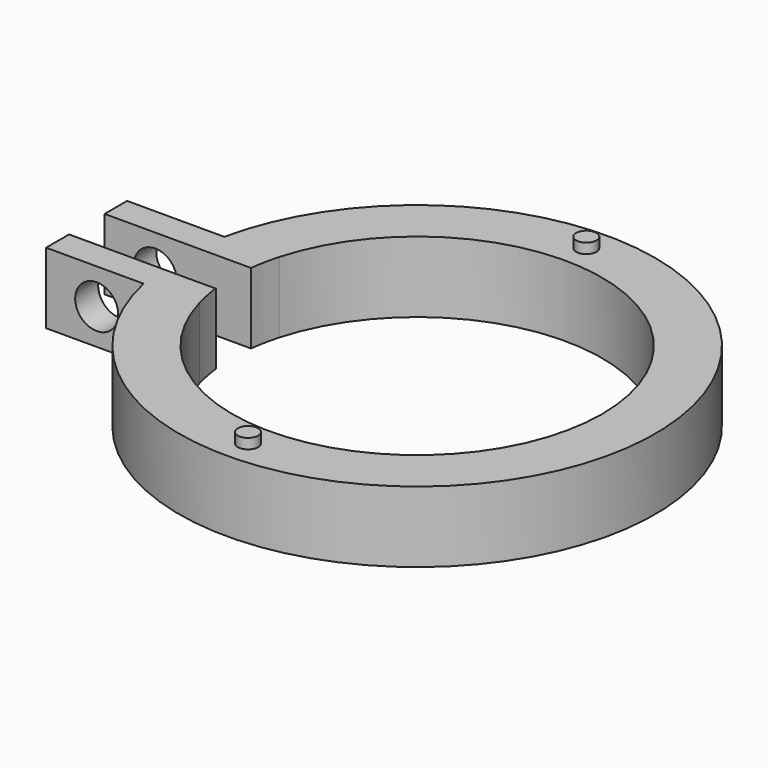
from build123d import *

# Parameters (mm, degrees)
F1_DEPTH = 7
F2_R     = 2.125
F3_DEPTH = 10
F4_R     = 1
F5_DEPTH = 1


# Not quite as in the source:
# - a feature names something its author has since deleted; it is built from what else it names


with BuildPart() as f1:
    # F0 (on Top) → F1 (new body)
    with BuildSketch(Plane.XY):
        with BuildLine():
            ThreePointArc((-23.401635828, 2.1478921234), (-23.2315061267, 3.5421918479), (-22.9783775489, 4.9238364331))
            Line((-22.9783775489, 4.9238364331), (-32.5732277849, 4.9238364331))
            Line((-32.5732277849, 4.9238364331), (-32.5732277849, 2.1478921234))
            Line((-32.5732277849, 2.1478921234), (-23.401635828, 2.1478921234))
        make_face()
        with BuildLine():
            Line((-32.5732277849, -5.0761635669), (-22.9452078535, -5.0761635669))
            ThreePointArc((-22.9452078535, -5.0761635669), (-23.2124017724, -3.6652972535), (-23.3929275249, -2.2407458164))
            Line((-23.3929275249, -2.2407458164), (-32.5732277849, -2.2407458164))
            Line((-32.5732277849, -2.2407458164), (-32.5732277849, -5.0761635669))
        make_face()
        with BuildLine():
            ThreePointArc((-22.9452078535, -5.0761635669), (2.55319559, -23.3608902287), (23.5, 0))
            ThreePointArc((23.5, 0), (2.4756946097, 23.3692305436), (-22.9783775489, 4.9238364331))
            Line((-22.9783775489, 4.9238364331), (-17.5732277849, 4.9238364331))
            ThreePointArc((-17.5732277849, 4.9238364331), (2.4850646798, 18.080015308), (18.25, 0))
            ThreePointArc((18.25, 0), (2.4850646798, -18.080015308), (-17.5732277849, -4.9238364331))
            Line((-17.5732277849, -4.9238364331), (-17.5732277849, -5.0761635669))
            Line((-17.5732277849, -5.0761635669), (-22.9452078535, -5.0761635669))
        make_face()
        with BuildLine():
            Line((-17.5732277849, 4.9238364331), (-22.9783775489, 4.9238364331))
            ThreePointArc((-22.9783775489, 4.9238364331), (-23.2315061267, 3.5421918479), (-23.401635828, 2.1478921234))
            Line((-23.401635828, 2.1478921234), (-18.1231636153, 2.1478921234))
            ThreePointArc((-18.1231636153, 2.1478921234), (-17.9020824613, 3.5465396584), (-17.5732277849, 4.9238364331))
        make_face()
        with BuildLine():
            ThreePointArc((-23.3929275249, -2.2407458164), (-23.2124017724, -3.6652972535), (-22.9452078535, -5.0761635669))
            Line((-22.9452078535, -5.0761635669), (-17.5732277849, -5.0761635669))
            Line((-17.5732277849, -5.0761635669), (-17.5732277849, -4.9238364331))
            ThreePointArc((-17.5732277849, -4.9238364331), (-17.9020824613, -3.5465396584), (-18.1231636153, -2.1478921234))
            Line((-18.1231636153, -2.1478921234), (-18.1231636153, -2.2407458164))
            Line((-18.1231636153, -2.2407458164), (-23.3929275249, -2.2407458164))
        make_face()
    extrude(amount=F1_DEPTH)

    # F2 (on face) → F3 (cut)
    with BuildSketch(Plane.XZ.offset(5.0761635669)):
        with Locations((-27.5732277849, 3.5)):
            Circle(F2_R)
    extrude(amount=-F3_DEPTH, mode=Mode.SUBTRACT)

    # F4 (on face) → F5 (join, symmetric)
    with BuildSketch(Plane.XY.offset(7)):
        with Locations((0, -20.875)):
            Circle(F4_R)
        with Locations((0, 20.875)):
            Circle(F4_R)
    extrude(amount=F5_DEPTH, both=True)


solid = f1.part
